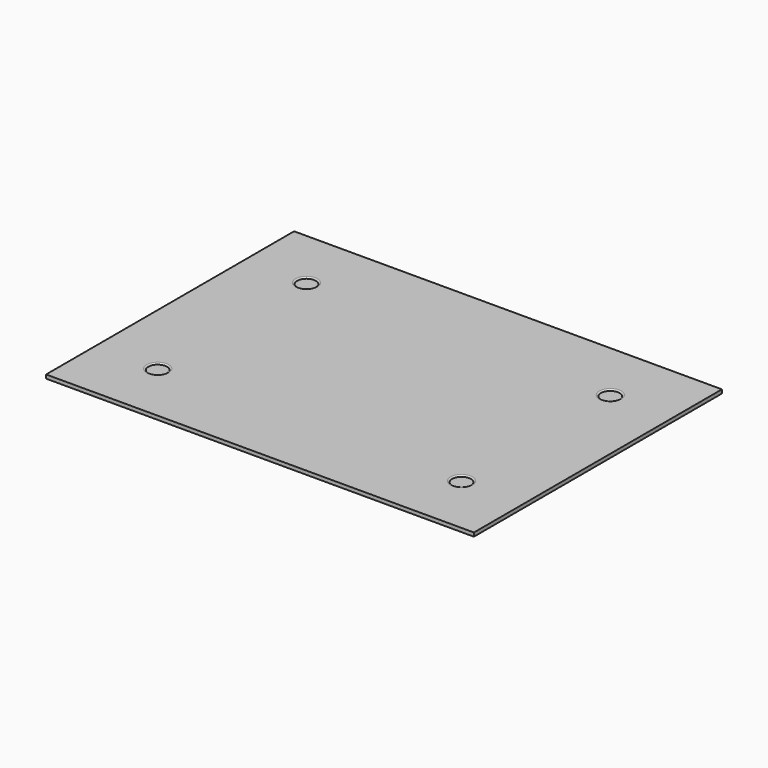
from build123d import *

# Parameters (mm, degrees)
F0_W     = 345
F0_H     = 250
F1_DEPTH = 3
F2_R     = 7.5
F3_DEPTH = 1


# Not quite as in the source:
# - a fillet or chamfer that OpenCascade refuses, or shapes differently, is made with other operations: its cross-section is extruded or revolved along the edge and cut away or added


with BuildPart() as f1:
    # F0 (on Top) → F1 (new body)
    with BuildSketch(Plane.XY):
        Rectangle(F0_W, F0_H)
    extrude(amount=F1_DEPTH)

    # F2 (on face) → F3 (cut)
    with BuildSketch(Plane.XY.offset(3)):
        with BuildLine():
            Line((-122.5, 75), (-122.5, 82.5))
            ThreePointArc((-122.5, 82.5), (-127.8033008589, 80.3033008589), (-130, 75))
            Line((-130, 75), (-122.5, 75))
        make_face()
        with BuildLine():
            ThreePointArc((-115, 75), (-117.1966991411, 80.3033008589), (-122.5, 82.5))
            Line((-122.5, 82.5), (-122.5, 75))
            Line((-122.5, 75), (-130, 75))
            ThreePointArc((-130, 75), (-122.5, 67.5), (-115, 75))
        make_face()
        with Locations((122.5, 75)):
            Circle(F2_R)
        with Locations((122.5, -75)):
            Circle(F2_R)
        with Locations((-122.5, -75)):
            Circle(F2_R)
    extrude(amount=-F3_DEPTH, mode=Mode.SUBTRACT)

    # F4: fillet of radius 1.5 on 4 edges, made by hand

    # F4_s1 → F4_t2 (revolve, cut)
    with BuildSketch(Plane.XZ.offset(-75)):
        with BuildLine():
            ThreePointArc((-131.4142135624, 3), (-130.5481881586, 2.7247448714), (-130, 2))
            Line((-130, 2), (-130, 3))
            Line((-130, 3), (-131.4142135624, 3))
        make_face()
    revolve(axis=Axis((-122.5, 75, 3), (0, 0, 1)), mode=Mode.SUBTRACT)

    # F4_s3 → F4_t4 (revolve, cut)
    with BuildSketch(Plane.XZ.offset(75)):
        with BuildLine():
            ThreePointArc((-113.5857864376, 3), (-114.4518118414, 2.7247448714), (-115, 2))
            Line((-115, 2), (-115, 3))
            Line((-115, 3), (-113.5857864376, 3))
        make_face()
    revolve(axis=Axis((-122.5, -75, 3), (0, 0, 1)), mode=Mode.SUBTRACT)

    # F4_s5 → F4_t6 (revolve, cut)
    with BuildSketch(Plane.XZ.offset(75)):
        with BuildLine():
            ThreePointArc((131.4142135624, 3), (130.5481881586, 2.7247448714), (130, 2))
            Line((130, 2), (130, 3))
            Line((130, 3), (131.4142135624, 3))
        make_face()
    revolve(axis=Axis((122.5, -75, 3), (0, 0, 1)), mode=Mode.SUBTRACT)

    # F4_s7 → F4_t8 (revolve, cut)
    with BuildSketch(Plane.XZ.offset(-75)):
        with BuildLine():
            ThreePointArc((131.4142135624, 3), (130.5481881586, 2.7247448714), (130, 2))
            Line((130, 2), (130, 3))
            Line((130, 3), (131.4142135624, 3))
        make_face()
    revolve(axis=Axis((122.5, 75, 3), (0, 0, 1)), mode=Mode.SUBTRACT)


solid = f1.part
